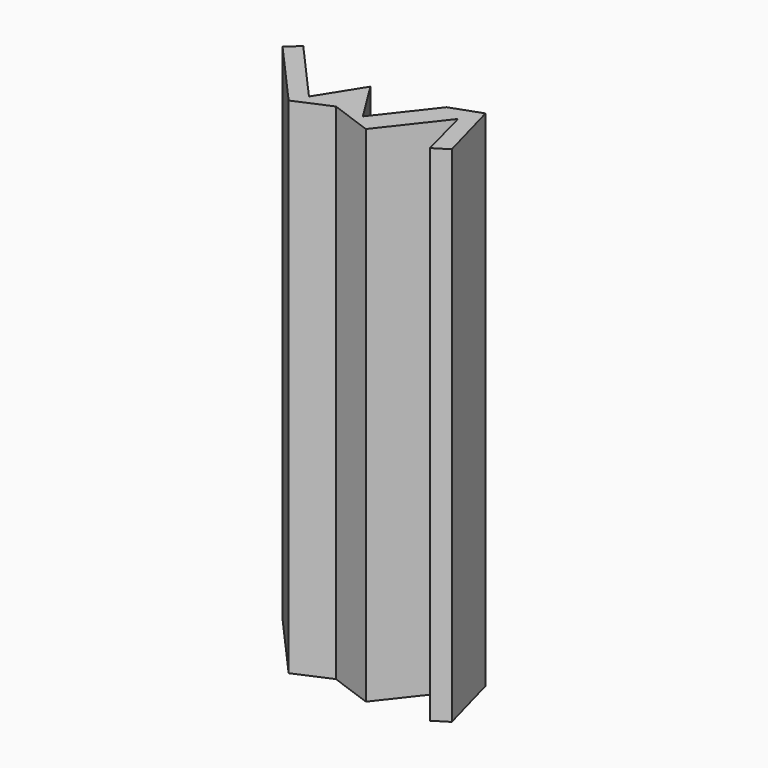
from build123d import *

# Parameters (mm, degrees)
F1_DEPTH = 304.8


# Not quite as in the source:
# - ends of sketch curves that miss each other by under 0.0002 mm in the source are joined


with BuildPart() as f1:
    # F0 (on Top) → F1 (new body)
    with BuildSketch(Plane.XY):
        Polygon((-62.3285062611, 56.3197806478), (-69.653712213, 49.8079545796), (-32.9701814049, 8.5423532873), (-11.6964066401, 17.7460387565), (13.72712516, 8.5423532873), (41.2449611033, 43.7803976238), (49.5065115392, 12.2516211122), (58.3160184324, 17.7460387565), (47.8142945757, 56.3197806478), (29.5691974461, 49.8079545796), (4.5316405594, 17.7460387565), (-11.6964066401, 43.7803976238), (-28.0378172673, 17.7460387565), align=None)
    extrude(amount=F1_DEPTH)


solid = f1.part
